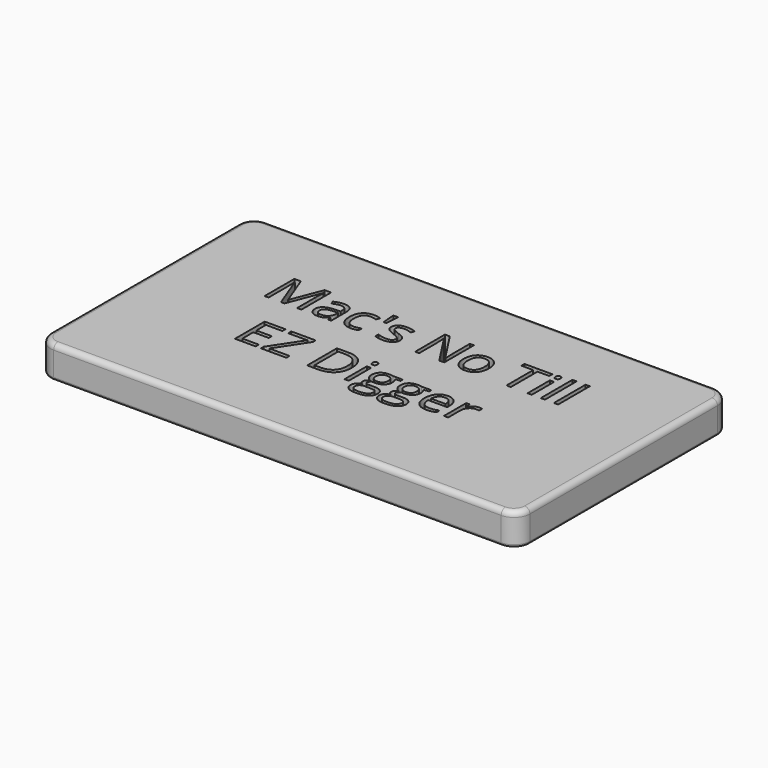
from build123d import *

# Parameters (mm, degrees)
F0_W         = 90
F0_H         = 50
F1_DEPTH     = 6
F2_R         = 1
F3_R         = 0.5
F4_T1_DEPTH  = 6
F4_T4_ANGLE  = 90
F4_T6_ANGLE  = 90
F4_T8_ANGLE  = 90
F4_T10_ANGLE = 90
F4_T12_ANGLE = 90
F4_T14_ANGLE = 90
F4_T16_ANGLE = 90
F4_T18_ANGLE = 90
F5_TEXT_SIZE = 9.7736017779
F6_DEPTH     = 6.0010001


# Not quite as in the source:
# - a fillet or chamfer that OpenCascade refuses, or shapes differently, is made with other operations: its cross-section is extruded or revolved along the edge and cut away or added
# - Text() gives the source's letters only with a copy of the font that has no kerning and outlines rounded to 1/6400 em; it was checked with that copy


with BuildPart() as f1:
    # F0 (on Top) → F1 (new body)
    with BuildSketch(Plane.XY):
        Rectangle(F0_W, F0_H)
    extrude(amount=-F1_DEPTH)

    # F2
    f2_edges = [f1.edges().sort_by_distance(p)[0] for p in [
        (45, 0, 0),
        (0, 25, 0),
        (-45, 0, 0),
        (0, -25, 0),
    ]]
    fillet(f2_edges, radius=F2_R)

    # F3
    f3_edges = [f1.edges().sort_by_distance(p)[0] for p in [
        (45, 0, -6),
        (0, 25, -6),
        (-45, 0, -6),
        (0, -25, -6),
    ]]
    fillet(f3_edges, radius=F3_R)

    # F4: fillet of radius 3 on 4 edges, made by hand

    # F4_s2 → F4_t1 (cut)
    with BuildSketch(Plane.XY.offset(-6)):
        with BuildLine():
            ThreePointArc((-42, -25), (-44.1213203436, -24.1213203436), (-45, -22))
            Line((-45, -22), (-45, -25))
            Line((-45, -25), (-42, -25))
        make_face()
        with BuildLine():
            ThreePointArc((45, -22), (44.1213203436, -24.1213203436), (42, -25))
            Line((42, -25), (45, -25))
            Line((45, -25), (45, -22))
        make_face()
        with BuildLine():
            ThreePointArc((-42, 25), (-44.1213203436, 24.1213203436), (-45, 22))
            Line((-45, 22), (-45, 25))
            Line((-45, 25), (-42, 25))
        make_face()
        with BuildLine():
            ThreePointArc((45, 22), (44.1213203436, 24.1213203436), (42, 25))
            Line((42, 25), (45, 25))
            Line((45, 25), (45, 22))
        make_face()
    extrude(amount=F4_T1_DEPTH, mode=Mode.SUBTRACT)

    # F4_s3 → F4_t4 (revolve, cut)
    with BuildSketch(Plane.XZ.offset(-22)):
        with BuildLine():
            ThreePointArc((44, 0), (44.7071067812, -0.2928932188), (45, -1))
            Line((45, -1), (45, 0))
            Line((45, 0), (44, 0))
        make_face()
    revolve(axis=Axis((42, 22, 0), (0, 0, 1)), revolution_arc=F4_T4_ANGLE, mode=Mode.SUBTRACT)

    # F4_s5 → F4_t6 (revolve, cut)
    with BuildSketch(Plane.YZ.offset(42)):
        with BuildLine():
            ThreePointArc((24.5, -6), (24.8535533906, -5.8535533906), (25, -5.5))
            Line((25, -5.5), (25, -6))
            Line((25, -6), (24.5, -6))
        make_face()
    revolve(axis=Axis((42, 22, -6), (0, 0, -1)), revolution_arc=F4_T6_ANGLE, mode=Mode.SUBTRACT)

    # F4_s7 → F4_t8 (revolve, cut)
    with BuildSketch(Plane.YZ.offset(-42)):
        with BuildLine():
            ThreePointArc((24, 0), (24.7071067812, -0.2928932188), (25, -1))
            Line((25, -1), (25, 0))
            Line((25, 0), (24, 0))
        make_face()
    revolve(axis=Axis((-42, 22, 0), (0, 0, 1)), revolution_arc=F4_T8_ANGLE, mode=Mode.SUBTRACT)

    # F4_s9 → F4_t10 (revolve, cut)
    with BuildSketch(Plane.XZ.offset(-22)):
        with BuildLine():
            ThreePointArc((-44.5, -6), (-44.8535533906, -5.8535533906), (-45, -5.5))
            Line((-45, -5.5), (-45, -6))
            Line((-45, -6), (-44.5, -6))
        make_face()
    revolve(axis=Axis((-42, 22, -6), (0, 0, -1)), revolution_arc=F4_T10_ANGLE, mode=Mode.SUBTRACT)

    # F4_s11 → F4_t12 (revolve, cut)
    with BuildSketch(Plane.YZ.offset(42)):
        with BuildLine():
            ThreePointArc((-24, 0), (-24.7071067812, -0.2928932188), (-25, -1))
            Line((-25, -1), (-25, 0))
            Line((-25, 0), (-24, 0))
        make_face()
    revolve(axis=Axis((42, -22, 0), (0, 0, 1)), revolution_arc=F4_T12_ANGLE, mode=Mode.SUBTRACT)

    # F4_s13 → F4_t14 (revolve, cut)
    with BuildSketch(Plane.XZ.offset(22)):
        with BuildLine():
            ThreePointArc((44.5, -6), (44.8535533906, -5.8535533906), (45, -5.5))
            Line((45, -5.5), (45, -6))
            Line((45, -6), (44.5, -6))
        make_face()
    revolve(axis=Axis((42, -22, -6), (0, 0, -1)), revolution_arc=F4_T14_ANGLE, mode=Mode.SUBTRACT)

    # F4_s15 → F4_t16 (revolve, cut)
    with BuildSketch(Plane.XZ.offset(22)):
        with BuildLine():
            ThreePointArc((-44, 0), (-44.7071067812, -0.2928932188), (-45, -1))
            Line((-45, -1), (-45, 0))
            Line((-45, 0), (-44, 0))
        make_face()
    revolve(axis=Axis((-42, -22, 0), (0, 0, 1)), revolution_arc=F4_T16_ANGLE, mode=Mode.SUBTRACT)

    # F4_s17 → F4_t18 (revolve, cut)
    with BuildSketch(Plane.YZ.offset(-42)):
        with BuildLine():
            ThreePointArc((-24.5, -6), (-24.8535533906, -5.8535533906), (-25, -5.5))
            Line((-25, -5.5), (-25, -6))
            Line((-25, -6), (-24.5, -6))
        make_face()
    revolve(axis=Axis((-42, -22, -6), (0, 0, -1)), revolution_arc=F4_T18_ANGLE, mode=Mode.SUBTRACT)

    # F5 (on face) → F6 (cut, through all)
    with BuildSketch(Plane.XY):
        with Locations((-28.3533714701, 6.2160990201)):
            Text("Mac's No Till", F5_TEXT_SIZE, font='Open Sans', text_align=(TextAlign.LEFT, TextAlign.BOTTOM))
        with Locations((-23.2741527961, -7.0759993978)):
            Text('EZ Digger', F5_TEXT_SIZE, font='Open Sans', text_align=(TextAlign.LEFT, TextAlign.BOTTOM))
    extrude(amount=-F6_DEPTH, mode=Mode.SUBTRACT)


solid = f1.part
